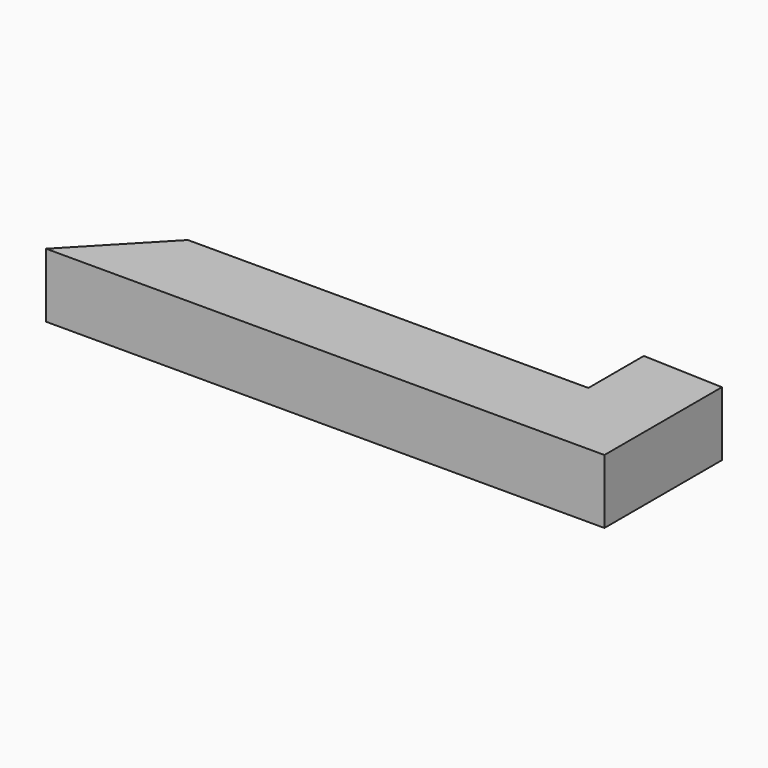
from build123d import *

# Parameters (mm, degrees)
F1_DEPTH = 13
F3_REACH = 70.401
F5_REACH = 197.0178690716
F7_DEPTH = 14.5
F8_W     = 6.5
F8_H     = 7
F9_DEPTH = 2


with BuildPart() as f1:
    # F0 (on Top) → F1 (new body)
    with BuildSketch(Plane.XY):
        Polygon((-43.3400757611, 0), (0, 0), (0, 45.5), (-22.9823845586, 46.4), (-22.9823845586, 23), (-150.9823845586, 23), (-173, 0), align=None)
    extrude(amount=-F1_DEPTH)

    f3_end = Plane(origin=(-11.4911922793, 45.95, -6.5), x_dir=(0.9992341112, -0.0391304348, 0), z_dir=(0.0391304348, 0.9992341112, 0))
    # F2 (on face) → F3 (join, up to a plane its end follows)
    with BuildSketch(Plane.XZ):
        Polygon((-20.9823845586, -13), (-22.9823845586, -13), (0, -19.9144775652), (0, -13), align=None)
    f3_long = extrude(amount=-F3_REACH, mode=Mode.PRIVATE)
    add(split(f3_long, bisect_by=f3_end, keep=Keep.BOTTOM, mode=Mode.PRIVATE))

    f5_end = Plane(origin=(-161.9911922793, 11.5, -6.5), x_dir=(-0.6915115049, -0.7223654467, 0), z_dir=(-0.7223654467, 0.6915115049, 0))
    # F4 (on face) → F5 (join, up to a plane its end follows)
    with BuildSketch(Plane.YZ):
        Polygon((23, -13), (0, -13), (0, -19.9144775652), align=None)
    f5_long = extrude(amount=-F5_REACH, mode=Mode.PRIVATE)
    add(split(f5_long, bisect_by=f5_end, keep=Keep.BOTTOM, mode=Mode.PRIVATE))

    # F6 (on face) → F7 (join)
    with BuildSketch(Plane.XY):
        Polygon((-149.0678093028, 25), (-150.9823845586, 23), (-22.9823845586, 23), (-22.9823845586, 46.4), (-24.9823845586, 46.4783208546), (-24.9823845586, 25), align=None)
    extrude(amount=-F7_DEPTH)

    # F8 (on face) → F9 (cut)
    with BuildSketch(Plane(origin=(0, 25, 0), x_dir=(-1, 0, 0), z_dir=(0, 1, 0))):
        with Locations((143.8178093028, -5.5)):
            Rectangle(F8_W, F8_H)
        with BuildLine():
            ThreePointArc((140.5678093028, -9), (143.8178093028, -12.25), (147.0678093028, -9))
            Line((147.0678093028, -9), (140.5678093028, -9))
        make_face()
        with BuildLine():
            Line((139.0678093028, -9), (132.5678093028, -9))
            ThreePointArc((132.5678093028, -9), (135.8178093028, -12.25), (139.0678093028, -9))
        make_face()
        with Locations((135.8178093028, -5.5)):
            Rectangle(F8_W, F8_H)
        with Locations((127.8178093028, -5.5)):
            Rectangle(F8_W, F8_H)
        with Locations((119.8178093028, -5.5)):
            Rectangle(F8_W, F8_H)
        with Locations((111.8178093028, -5.5)):
            Rectangle(F8_W, F8_H)
        with Locations((103.8178093028, -5.5)):
            Rectangle(F8_W, F8_H)
        with Locations((95.8178093028, -5.5)):
            Rectangle(F8_W, F8_H)
        with Locations((87.8178093028, -5.5)):
            Rectangle(F8_W, F8_H)
        with Locations((79.8178093028, -5.5)):
            Rectangle(F8_W, F8_H)
        with Locations((71.8178093028, -5.5)):
            Rectangle(F8_W, F8_H)
        with Locations((63.8178093028, -5.5)):
            Rectangle(F8_W, F8_H)
        with Locations((55.8178093028, -5.5)):
            Rectangle(F8_W, F8_H)
        with Locations((47.8178093028, -5.5)):
            Rectangle(F8_W, F8_H)
        with Locations((39.8178093028, -5.5)):
            Rectangle(F8_W, F8_H)
        with Locations((31.8178093028, -5.5)):
            Rectangle(F8_W, F8_H)
        with BuildLine():
            Line((35.0678093028, -9), (28.5678093028, -9))
            ThreePointArc((28.5678093028, -9), (31.8178093028, -12.25), (35.0678093028, -9))
        make_face()
        with BuildLine():
            Line((43.0678093028, -9), (36.5678093028, -9))
            ThreePointArc((36.5678093028, -9), (39.8178093028, -12.25), (43.0678093028, -9))
        make_face()
        with BuildLine():
            Line((51.0678093028, -9), (44.5678093028, -9))
            ThreePointArc((44.5678093028, -9), (47.8178093028, -12.25), (51.0678093028, -9))
        make_face()
        with BuildLine():
            Line((59.0678093028, -9), (52.5678093028, -9))
            ThreePointArc((52.5678093028, -9), (55.8178093028, -12.25), (59.0678093028, -9))
        make_face()
        with BuildLine():
            Line((67.0678093028, -9), (60.5678093028, -9))
            ThreePointArc((60.5678093028, -9), (63.8178093028, -12.25), (67.0678093028, -9))
        make_face()
        with BuildLine():
            Line((75.0678093028, -9), (68.5678093028, -9))
            ThreePointArc((68.5678093028, -9), (71.8178093028, -12.25), (75.0678093028, -9))
        make_face()
        with BuildLine():
            Line((83.0678093028, -9), (76.5678093028, -9))
            ThreePointArc((76.5678093028, -9), (79.8178093028, -12.25), (83.0678093028, -9))
        make_face()
        with BuildLine():
            Line((91.0678093028, -9), (84.5678093028, -9))
            ThreePointArc((84.5678093028, -9), (87.8178093028, -12.25), (91.0678093028, -9))
        make_face()
        with BuildLine():
            Line((99.0678093028, -9), (92.5678093028, -9))
            ThreePointArc((92.5678093028, -9), (95.8178093028, -12.25), (99.0678093028, -9))
        make_face()
        with BuildLine():
            Line((107.0678093028, -9), (100.5678093028, -9))
            ThreePointArc((100.5678093028, -9), (103.8178093028, -12.25), (107.0678093028, -9))
        make_face()
        with BuildLine():
            Line((115.0678093028, -9), (108.5678093028, -9))
            ThreePointArc((108.5678093028, -9), (111.8178093028, -12.25), (115.0678093028, -9))
        make_face()
        with BuildLine():
            Line((123.0678093028, -9), (116.5678093028, -9))
            ThreePointArc((116.5678093028, -9), (119.8178093028, -12.25), (123.0678093028, -9))
        make_face()
        with BuildLine():
            Line((131.0678093028, -9), (124.5678093028, -9))
            ThreePointArc((124.5678093028, -9), (127.8178093028, -12.25), (131.0678093028, -9))
        make_face()
    extrude(amount=-F9_DEPTH, mode=Mode.SUBTRACT)


solid = f1.part
